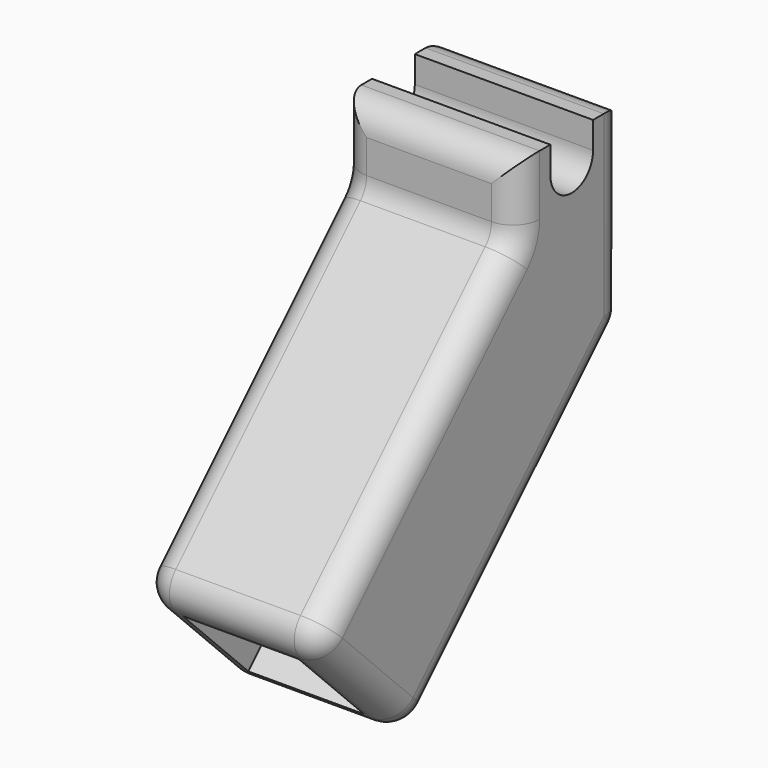
from build123d import *

# Parameters (mm, degrees)
F1_DEPTH    = 20
F2_W        = 13
F2_H        = 13
F3_DEPTH    = 40
F4_R        = 2.5
F5_REACH    = 22.0720678119
F6_F1_R     = 3
F6_F2_R     = 3
F7_DEPTH    = 3
F8_T1_DEPTH = 29


# Not quite as in the source:
# - a fillet or chamfer that OpenCascade refuses, or shapes differently, is made with other operations: its cross-section is extruded or revolved along the edge and cut away or added


with BuildPart() as f1:
    # F0 (on Right) → F1 (new body)
    with BuildSketch(Plane.YZ):
        with BuildLine():
            Line((0, -18.2842712475), (0, 0))
            Line((0, 0), (-4.5, 0))
            ThreePointArc((-4.5, 0), (-7.5, -3), (-10.5, 0))
            Line((-10.5, 0), (-15, 0))
            Line((-15, 0), (-15, -5))
            Line((-15, -5), (-43.8908729653, -33.8908729653))
            Line((-43.8908729653, -33.8908729653), (-29.7487373415, -48.033008589))
            Line((-29.7487373415, -48.033008589), (0, -18.2842712475))
        make_face()
    extrude(amount=F1_DEPTH)

    # F2 (on face) → F3 (cut)
    with BuildSketch(Plane(origin=(0, -38.8908729653, -38.8908729653), x_dir=(1, 0, 0), z_dir=(0, -0.7071067812, -0.7071067812))):
        with Locations((10, -2.9289321881)):
            Rectangle(F2_W, F2_H)
    extrude(amount=-F3_DEPTH, mode=Mode.SUBTRACT)

    f5_end = f1.faces().sort_by_distance((10, 0, -9.1421356237))[0]
    # F4 (on face) → F5 (cut, up to a face of the model that its end follows)
    with BuildSketch(Plane(origin=(0, -10.6066017178, -10.6066017178), x_dir=(1, 0, 0), z_dir=(0, -0.7071067812, -0.7071067812))):
        with Locations((10, -2.9289321881)):
            Circle(F4_R)
    f5_long = extrude(amount=-F5_REACH, mode=Mode.PRIVATE)
    add(split(f5_long, bisect_by=f5_end, keep=Keep.BOTTOM, mode=Mode.PRIVATE), mode=Mode.SUBTRACT)

    # F6: fillet of radius 3 on 12 edges, made by hand

    # F6_f1
    f6_f1_edges = [f1.edges().sort_by_distance(p)[0] for p in [
        (10, -15, -5),
    ]]
    fillet(f6_f1_edges, radius=F6_F1_R)

    # F6_f2
    f6_f2_edges = [f1.edges().sort_by_distance(p)[0] for p in [
        (10, -43.8908729653, -33.8908729653),
        (0, -36.8198051534, -40.9619407771),
        (10, -29.7487373415, -48.033008589),
        (20, -36.8198051534, -40.9619407771),
        (10, 0, -18.2842712475),
        (20, -14.8743686708, -33.1586399182),
        (20, 0, -9.1421356237),
        (20, -15, -1.8786796564),
        (0, -15, -1.8786796564),
        (0, -14.8743686708, -33.1586399182),
        (0, 0, -9.1421356237),
        (0, -15.2283614025, -4.90540961),
        (20, -15.2283614025, -4.90540961),
    ]]
    fillet(f6_f2_edges, radius=F6_F2_R)

    # F7 (add): faces of the model
    f7_faces = [f1.faces().sort_by_distance(p)[0] for p in [
        (10, -2.3208506609, 0),
        (10, -12.6791493391, 0),
    ]]
    extrude(f7_faces, amount=F7_DEPTH)

    # F8: fillet of radius 3 on 2 edges, made by hand

    # F8_s2 → F8_t1 (cut)
    with BuildSketch(Plane.YZ.offset(-4.5)):
        with BuildLine():
            ThreePointArc((-15, 0), (-14.1213203436, 2.1213203436), (-12, 3))
            Line((-12, 3), (-15, 3))
            Line((-15, 3), (-15, 0))
        make_face()
        with BuildLine():
            ThreePointArc((-3, 3), (-0.8786796564, 2.1213203436), (0, 0))
            Line((0, 0), (0, 3))
            Line((0, 3), (-3, 3))
        make_face()
    extrude(amount=F8_T1_DEPTH, mode=Mode.SUBTRACT)


solid = f1.part
